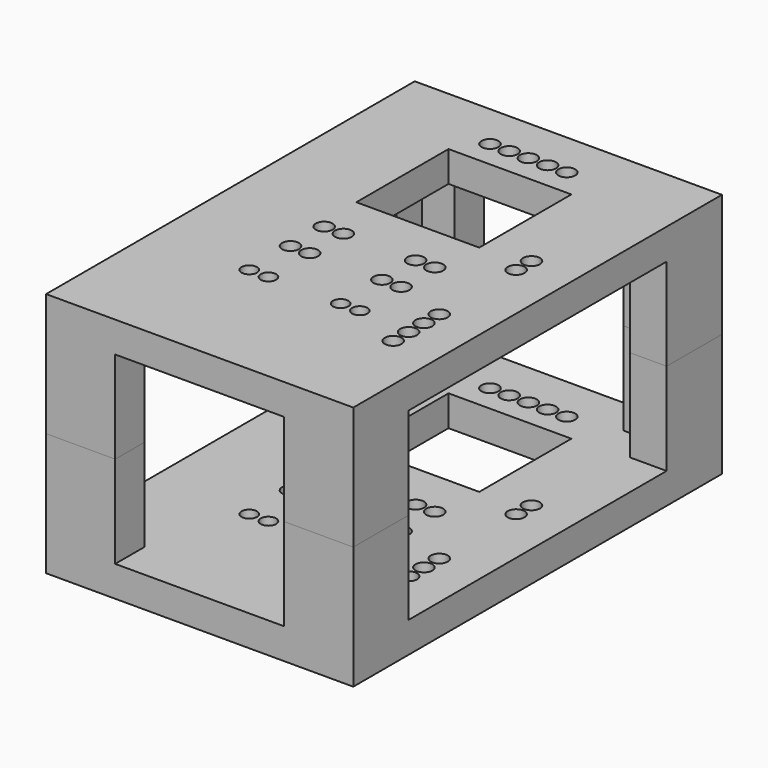
from build123d import *

# Parameters (mm, degrees)
F0_W     = 2.4
F0_H     = 21
F0_W_2   = 11
F0_H_2   = 2.4
F0_W_3   = 8
F0_H_3   = 7.5
F1_DEPTH = 2
F2_DEPTH = 6
F3_D     = 1.1
F4_D     = 1.1
F5_D     = 1


# Not quite as in the source:
# - a feature names something its author has since deleted; it is built from what else it names


with BuildPart() as f1:
    # F0 (on Top) → F1 (new body)
    with BuildSketch(Plane.XY):
        with Locations((-55.0351821041, -18.9141327012)):
            Rectangle(F0_W, F0_H)
        with Locations((-46.2351821041, -32.7141327012)):
            Rectangle(F0_W_2, F0_H_2)
        Polygon((-51.7351821041, -33.9141327012), (-51.7351821041, -31.5141327012), (-53.8351821041, -31.5141327012), (-53.8351821041, -29.4141327012), (-56.2351821041, -29.4141327012), (-56.2351821041, -33.9141327012), align=None)
        Polygon((-38.6351821041, -29.4141327012), (-38.6351821041, -31.5141327012), (-40.7351821041, -31.5141327012), (-40.7351821041, -33.9141327012), (-36.2351821041, -33.9141327012), (-36.2351821041, -29.4141327012), align=None)
        Polygon((-38.6351821041, -26.1641327012), (-38.6351821041, -29.4141327012), (-36.2351821041, -29.4141327012), (-36.2351821041, -8.4141327012), (-38.6351821041, -8.4141327012), (-38.6351821041, -15.1641327012), (-38.6351821041, -16.1641327012), (-38.6351821041, -16.4141327012), (-38.6351821041, -17.4141327012), (-38.6351821041, -22.6641327012), (-38.6351821041, -23.6641327012), (-38.6351821041, -23.9141327012), (-38.6351821041, -24.9141327012), (-38.6351821041, -25.1641327012), align=None)
        Polygon((-38.6351821041, -8.4141327012), (-36.2351821041, -8.4141327012), (-36.2351821041, -3.9141327012), (-40.7351821041, -3.9141327012), (-40.7351821041, -6.3141327012), (-38.6351821041, -6.3141327012), align=None)
        Polygon((-40.7351821041, -6.3141327012), (-40.7351821041, -3.9141327012), (-51.7351821041, -3.9141327012), (-51.7351821041, -6.3141327012), (-49.4351821041, -6.3141327012), (-48.4351821041, -6.3141327012), (-48.1851821041, -6.3141327012), (-47.1851821041, -6.3141327012), (-46.9351821041, -6.3141327012), (-45.9351821041, -6.3141327012), (-45.6851821041, -6.3141327012), (-44.6851821041, -6.3141327012), (-44.4351821041, -6.3141327012), (-43.4351821041, -6.3141327012), align=None)
        Polygon((-56.2351821041, -8.4141327012), (-53.8351821041, -8.4141327012), (-53.8351821041, -6.3141327012), (-51.7351821041, -6.3141327012), (-51.7351821041, -3.9141327012), (-56.2351821041, -3.9141327012), align=None)
        Polygon((-40.7351821041, -31.5141327012), (-38.6351821041, -31.5141327012), (-38.6351821041, -29.4141327012), (-38.6351821041, -26.1641327012), (-38.6351821041, -25.1641327012), (-38.6351821041, -24.9141327012), (-38.6351821041, -23.9141327012), (-38.6351821041, -23.6641327012), (-38.6351821041, -22.6641327012), (-38.6351821041, -17.4141327012), (-38.6351821041, -16.4141327012), (-38.6351821041, -16.1641327012), (-38.6351821041, -15.1641327012), (-38.6351821041, -8.4141327012), (-38.6351821041, -6.3141327012), (-40.7351821041, -6.3141327012), (-43.4351821041, -6.3141327012), (-44.4351821041, -6.3141327012), (-44.6851821041, -6.3141327012), (-45.6851821041, -6.3141327012), (-45.9351821041, -6.3141327012), (-46.9351821041, -6.3141327012), (-47.1851821041, -6.3141327012), (-48.1851821041, -6.3141327012), (-48.4351821041, -6.3141327012), (-49.4351821041, -6.3141327012), (-51.7351821041, -6.3141327012), (-53.8351821041, -6.3141327012), (-53.8351821041, -8.4141327012), (-53.8351821041, -29.4141327012), (-53.8351821041, -31.5141327012), (-51.7351821041, -31.5141327012), align=None)
        with Locations((-46.2351821041, -12.4141327012)):
            Rectangle(F0_W_3, F0_H_3, mode=Mode.SUBTRACT)
    extrude(amount=-F1_DEPTH)

    # F0 (on Top) → F2 (join)
    with BuildSketch(Plane.XY):
        Polygon((-56.2351821041, -8.4141327012), (-53.8351821041, -8.4141327012), (-53.8351821041, -6.3141327012), (-51.7351821041, -6.3141327012), (-51.7351821041, -3.9141327012), (-56.2351821041, -3.9141327012), align=None)
        Polygon((-38.6351821041, -8.4141327012), (-36.2351821041, -8.4141327012), (-36.2351821041, -3.9141327012), (-40.7351821041, -3.9141327012), (-40.7351821041, -6.3141327012), (-38.6351821041, -6.3141327012), align=None)
        Polygon((-38.6351821041, -29.4141327012), (-38.6351821041, -31.5141327012), (-40.7351821041, -31.5141327012), (-40.7351821041, -33.9141327012), (-36.2351821041, -33.9141327012), (-36.2351821041, -29.4141327012), align=None)
        Polygon((-51.7351821041, -33.9141327012), (-51.7351821041, -31.5141327012), (-53.8351821041, -31.5141327012), (-53.8351821041, -29.4141327012), (-56.2351821041, -29.4141327012), (-56.2351821041, -33.9141327012), align=None)
    extrude(amount=F2_DEPTH)

    # F3 (through all)
    with Locations(Plane.XY):
        with Locations((-39.2351821041, -24.4141327012), (-39.2351821041, -23.1641327012), (-39.2351821041, -16.9141327012), (-39.2351821041, -15.6641327012), (-43.9351821041, -6.9141327012), (-45.1851821041, -6.9141327012), (-46.4351821041, -6.9141327012), (-47.6851821041, -6.9141327012), (-48.9351821041, -6.9141327012), (-39.2351821041, -25.6641327012), (-39.2351821041, -26.9141327012)):
            Hole(F3_D / 2)

    # F4 (through all)
    with Locations(Plane.XY):
        with Locations((-49.8351821041, -19.2821994424), (-48.5851821041, -19.2821994424), (-43.8851821041, -19.2821994424), (-42.6351821041, -19.2821994424), (-49.8351821041, -22.0237951726), (-48.5851821041, -22.0237951726), (-43.8851821041, -22.0237951726), (-42.6351821041, -22.0237951726)):
            Hole(F4_D / 2)

    # F5 (through all)
    with Locations(Plane.XY):
        with Locations((-49.8351821041, -25.3798887134), (-48.5851821041, -25.3798887134), (-43.8851821041, -25.3798887134), (-42.6351821041, -25.3798887134)):
            Hole(F5_D / 2)


with BuildPart() as f6_1:
    # F6: instance of F1
    add(f1.part.mirror(Plane(origin=(-54.3192730132, -31.9982236102, 6), x_dir=(1, 0, 0), z_dir=(0, 0, 1))))


solid = Compound([f1.part, f6_1.part])
